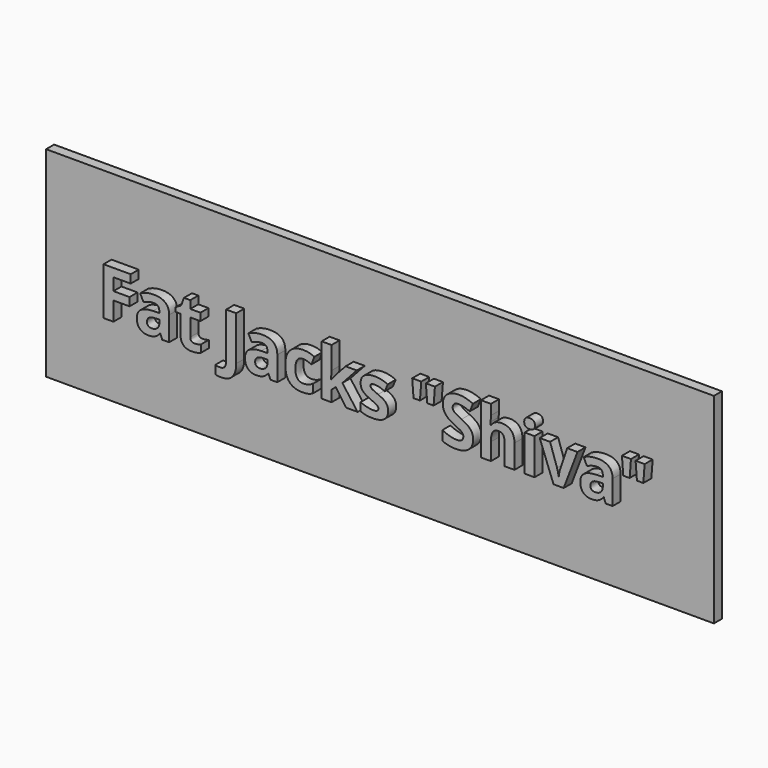
from build123d import *

# Parameters (mm, degrees)
F0_W         = 50
F0_H         = 30
F1_DEPTH     = 1.5
F2_TEXT_SIZE = 9.9429047113
F3_DEPTH     = 1.5


# Not quite as in the source:
# - Text() gives the source's letters only with a copy of the font that has no kerning and outlines rounded to 1/6400 em; it was checked with that copy


with BuildPart() as f1:
    # F0 (on Front) → F1 (new body)
    with BuildSketch(Plane.XZ):
        with Locations((25, 15)):
            Rectangle(F0_W, F0_H)
        with Locations((-25, 15)):
            Rectangle(F0_W, F0_H)
    extrude(amount=F1_DEPTH)

    # F2 (on face) → F3 (join)
    with BuildSketch(Plane.XZ.offset(1.5)):
        with Locations((-41.0882346332, 11.5341097116)):
            Text('Fat Jacks "Shiva"', F2_TEXT_SIZE, font='Open Sans', font_style=FontStyle.BOLD, text_align=(TextAlign.LEFT, TextAlign.BOTTOM))
    extrude(amount=F3_DEPTH)


solid = f1.part
